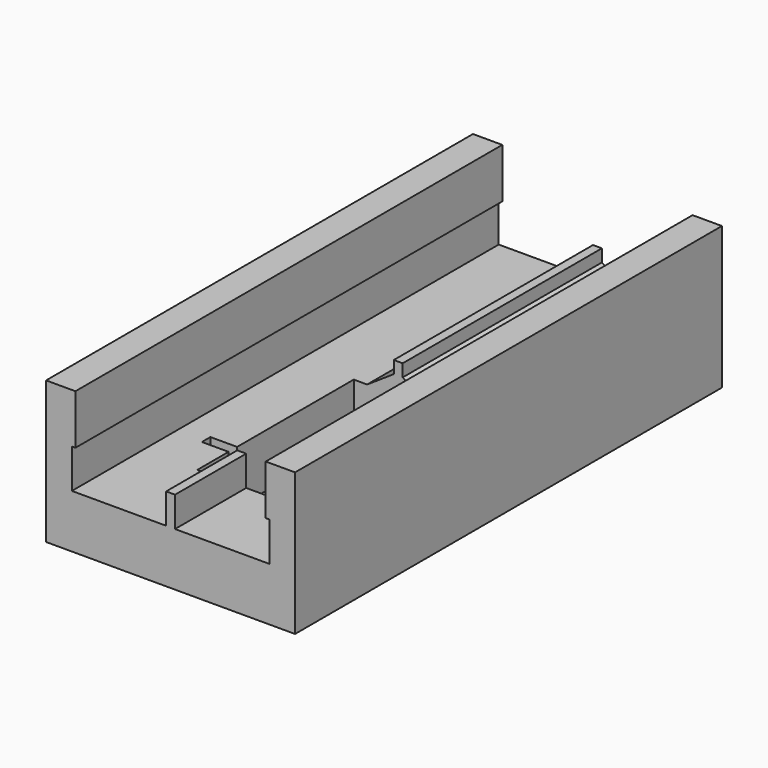
from build123d import *

# Parameters (mm, degrees)
F0_W     = 14
F0_H     = 8
F1_DEPTH = 30
F3_W     = 1.5
F3_H     = 0.6
F4_DEPTH = 8
F5_DEPTH = 30.001
F7_DEPTH = 5
F8_R     = 0.85
F9_DEPTH = 3


# Not quite as in the source:
# - a feature names something its author has since deleted; it is built from what else it names


with BuildPart() as f1:
    # F0 (on Front) → F1 (new body)
    with BuildSketch(Plane.XZ):
        Rectangle(F0_W, F0_H)
    extrude(amount=F1_DEPTH)

    # F3 (on face) → F4 (cut, through all)
    with BuildSketch(Plane(origin=(0, 0, -4), x_dir=(1, 0, 0), z_dir=(0, 0, -1))):
        with Locations((3.25, 22.5)):
            Rectangle(F3_W, F3_H)
        Polygon((-2.5, 14), (2.5, 14), (2.5, 22.2), (2.5, 22.8), (2.5, 25), (-2.5, 25), (-2.5, 22.8), (-2.5, 22.2), align=None)
        with Locations((-3.25, 22.5)):
            Rectangle(F3_W, F3_H)
    extrude(amount=-F4_DEPTH, mode=Mode.SUBTRACT)

    # F2 (on face) → F5 (cut, through all)
    with BuildSketch(Plane.XZ.offset(30)):
        Polygon((-0.25, 0), (-0.25, 0.7), (0.25, 0.7), (0.25, 0), (1.75, -1), (5.55, -1), (5.55, 1.2), (5.35, 1.2), (5.35, 4), (-5.35, 4), (-5.35, 1.2), (-5.55, 1.2), (-5.55, -1), (-1.75, -1), align=None)
    extrude(amount=-F5_DEPTH, mode=Mode.SUBTRACT)

    # F6 (on face) → F7 (cut, through all)
    with BuildSketch(Plane.XZ.offset(30)):
        Polygon((-0.25, -1), (-0.25, 0), (-1.75, -1), align=None)
        Polygon((1.75, -1), (0.25, 0), (0.25, -1), align=None)
    extrude(amount=-F7_DEPTH, mode=Mode.SUBTRACT)

    # F8 (on face) → F9 (cut)
    with BuildSketch(Plane(origin=(0, 0, -4), x_dir=(1, 0, 0), z_dir=(0, 0, -1))):
        with Locations((0, 7.5)):
            Circle(F8_R)
    extrude(amount=-F9_DEPTH, mode=Mode.SUBTRACT)


solid = f1.part
